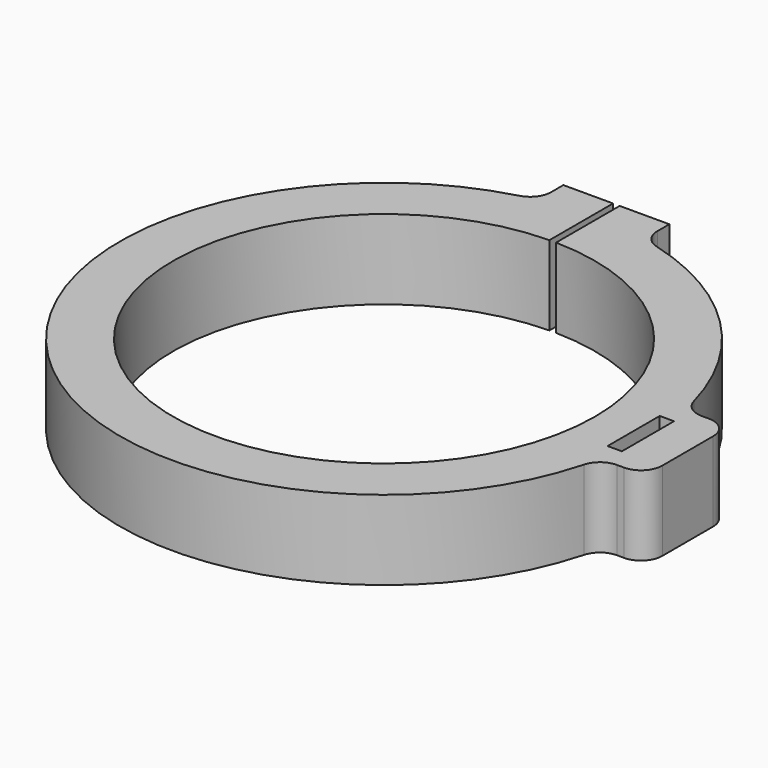
from build123d import *

# Parameters (mm, degrees)
F0_R          = 63.246
F0_R_2        = 50.546
F1_DEPTH      = 19.05
F3_DEPTH      = 19.05
F4_W          = 1.5875
F4_H          = 19.0562327178
F5_DEPTH      = 19.051
F6_R          = 2.5527
F7_DEPTH      = 11.90625
F8_R          = 5.1417133043
F9_DEPTH      = 3.175
F9_DEPTH_BACK = 50.547
F11_D         = 3.7973
F12_W         = 22.225
F12_H         = 25.4
F13_DEPTH     = 19.05
F14_W         = 3.429
F14_H         = 15.621
F15_DEPTH     = 19.0510001
F16_T1_DEPTH  = 19.05
F16_T6_DEPTH  = 14.4190086939
F16_S7_R      = 5.1417133043
F16_T8_DEPTH  = 9
F16_T12_DEPTH = 14.4190086939
F16_S13_R     = 5.1417133043
F16_T14_DEPTH = 9
F16_T18_DEPTH = 17.6620719982
F16_S19_R     = 1.89865
F16_T20_DEPTH = 11
F16_T24_DEPTH = 17.6620719982
F16_S25_R     = 1.89865
F16_T26_DEPTH = 11
F16_T27_DEPTH = 44.45


# Not quite as in the source:
# - a fillet or chamfer that OpenCascade refuses, or shapes differently, is made with other operations: its cross-section is extruded or revolved along the edge and cut away or added


with BuildPart() as f1:
    # F0 (on Top) → F1 (new body)
    with BuildSketch(Plane.XY):
        Circle(F0_R)
        Circle(F0_R_2, mode=Mode.SUBTRACT)
    extrude(amount=F1_DEPTH)

    # F2 (on face) → F3 (join)
    with BuildSketch(Plane.XY.offset(19.05)):
        with BuildLine():
            Line((12.7, 69.596), (-12.7, 69.596))
            Line((-12.7, 69.596), (-12.7, 61.9577801087))
            ThreePointArc((-12.7, 61.9577801087), (0, 63.246), (12.7, 61.9577801087))
            Line((12.7, 61.9577801087), (12.7, 69.596))
        make_face()
    extrude(amount=-F3_DEPTH)

    # F4 (on face) → F5 (cut, through all)
    with BuildSketch(Plane.XY.offset(19.05)):
        with Locations((0, 60.0678836411)):
            Rectangle(F4_W, F4_H)
    extrude(amount=-F5_DEPTH, mode=Mode.SUBTRACT)

    # F6 (on face) → F7 (cut, through all)
    with BuildSketch(Plane.YZ.offset(12.7)):
        with Locations((61.9577801087, 9.525)):
            Circle(F6_R)
    extrude(amount=-F7_DEPTH, mode=Mode.SUBTRACT)

    # F8 (on face) → F9 (cut, two sides)
    with BuildSketch(Plane.YZ.offset(12.7)) as f9_sk:
        with Locations((61.9577801087, 9.525)):
            Circle(F8_R)
    extrude(amount=-F9_DEPTH, mode=Mode.SUBTRACT)
    extrude(f9_sk.sketch, amount=F9_DEPTH_BACK, mode=Mode.SUBTRACT)

    # F11 (through all)
    with Locations(Plane.YZ.offset(-0.79375)):
        with Locations((61.9577801087, 9.525)):
            Hole(F11_D / 2)

    # F12 (on face) → F13 (join)
    with BuildSketch(Plane.XY.offset(19.05)):
        with Locations((61.6585, 0)):
            Rectangle(F12_W, F12_H)
    extrude(amount=-F13_DEPTH)

    # F14 (on face) → F15 (cut, through all)
    with BuildSketch(Plane.XY.offset(19.05)):
        with Locations((61.5315, 0)):
            Rectangle(F14_W, F14_H)
    extrude(amount=-F15_DEPTH, mode=Mode.SUBTRACT)

    # F16: fillet of radius 5.08 on 8 edges, made by hand

    # F16_s2 → F16_t1 (join)
    with BuildSketch(Plane.XY):
        with BuildLine():
            ThreePointArc((61.0670823721, -16.4580669145), (62.882491273, -13.7475181293), (65.972068908, -12.7))
            Line((65.972068908, -12.7), (61.9577801087, -12.7))
            ThreePointArc((61.9577801087, -12.7), (61.5411241678, -14.585833955), (61.0670823721, -16.4580669145))
        make_face()
        with BuildLine():
            ThreePointArc((65.972068908, 12.7), (62.882491273, 13.7475181293), (61.0670823721, 16.4580669145))
            ThreePointArc((61.0670823721, 16.4580669145), (61.5411241678, 14.585833955), (61.9577801087, 12.7))
            Line((61.9577801087, 12.7), (65.972068908, 12.7))
        make_face()
    extrude(amount=F16_T1_DEPTH)


with BuildPart() as f16_tool4:
    # F16_s5 → F16_t6 (new body)
    with BuildSketch(Plane.XY.offset(19.05)):
        with BuildLine():
            ThreePointArc((16.4580669145, 61.0670823721), (13.7475181293, 62.882491273), (12.7, 65.972068908))
            Line((12.7, 65.972068908), (12.7, 61.9577801087))
            ThreePointArc((12.7, 61.9577801087), (14.585833955, 61.5411241678), (16.4580669145, 61.0670823721))
        make_face()
    extrude(amount=-F16_T6_DEPTH)

    # F16_s7 → F16_t8 (cut, symmetric)
    with BuildSketch(Plane.YZ.offset(14.6)):
        with Locations((61.9577801087, 9.525)):
            Circle(F16_S7_R)
    extrude(amount=F16_T8_DEPTH, both=True, mode=Mode.SUBTRACT)


with BuildPart() as f1_1:
    add(f1.part)

    # F16_t3: union F16_tool4
    add(f16_tool4.part)


with BuildPart() as f16_tool10:
    # F16_s11 → F16_t12 (new body)
    with BuildSketch(Plane.XY.offset(14.4190086939)):
        with BuildLine():
            ThreePointArc((16.4580669145, 61.0670823721), (13.7475181293, 62.882491273), (12.7, 65.972068908))
            Line((12.7, 65.972068908), (12.7, 61.9577801087))
            ThreePointArc((12.7, 61.9577801087), (14.585833955, 61.5411241678), (16.4580669145, 61.0670823721))
        make_face()
    extrude(amount=-F16_T12_DEPTH)

    # F16_s13 → F16_t14 (cut, symmetric)
    with BuildSketch(Plane.YZ.offset(14.6)):
        with Locations((61.9577801087, 9.525)):
            Circle(F16_S13_R)
    extrude(amount=F16_T14_DEPTH, both=True, mode=Mode.SUBTRACT)


with BuildPart() as f1_2:
    add(f1_1.part)

    # F16_t9: union F16_tool10
    add(f16_tool10.part)


with BuildPart() as f16_tool16:
    # F16_s17 → F16_t18 (new body)
    with BuildSketch(Plane.XY.offset(19.05)):
        with BuildLine():
            ThreePointArc((-16.4580669145, 61.0670823721), (-13.7475181293, 62.882491273), (-12.7, 65.972068908))
            Line((-12.7, 65.972068908), (-12.7, 61.9577801087))
            ThreePointArc((-12.7, 61.9577801087), (-14.585833955, 61.5411241678), (-16.4580669145, 61.0670823721))
        make_face()
    extrude(amount=-F16_T18_DEPTH)

    # F16_s19 → F16_t20 (cut, symmetric)
    with BuildSketch(Plane.YZ.offset(-14.6)):
        with Locations((61.9577801087, 9.525)):
            Circle(F16_S19_R)
    extrude(amount=F16_T20_DEPTH, both=True, mode=Mode.SUBTRACT)


with BuildPart() as f1_3:
    add(f1_2.part)

    # F16_t15: union F16_tool16
    add(f16_tool16.part)


with BuildPart() as f16_tool22:
    # F16_s23 → F16_t24 (new body)
    with BuildSketch(Plane.XY.offset(17.6620719982)):
        with BuildLine():
            ThreePointArc((-16.4580669145, 61.0670823721), (-13.7475181293, 62.882491273), (-12.7, 65.972068908))
            Line((-12.7, 65.972068908), (-12.7, 61.9577801087))
            ThreePointArc((-12.7, 61.9577801087), (-14.585833955, 61.5411241678), (-16.4580669145, 61.0670823721))
        make_face()
    extrude(amount=-F16_T24_DEPTH)

    # F16_s25 → F16_t26 (cut, symmetric)
    with BuildSketch(Plane.YZ.offset(-14.6)):
        with Locations((61.9577801087, 9.525)):
            Circle(F16_S25_R)
    extrude(amount=F16_T26_DEPTH, both=True, mode=Mode.SUBTRACT)


with BuildPart() as f1_4:
    add(f1_3.part)

    # F16_t21: union F16_tool22
    add(f16_tool22.part)

    # F16_s28 → F16_t27 (cut)
    with BuildSketch(Plane.XY.offset(-12.7)):
        with BuildLine():
            ThreePointArc((67.691, -12.7), (71.2831024484, -11.2121024484), (72.771, -7.62))
            Line((72.771, -7.62), (72.771, -12.7))
            Line((72.771, -12.7), (67.691, -12.7))
        make_face()
        with BuildLine():
            ThreePointArc((72.771, 7.62), (71.2831024484, 11.2121024484), (67.691, 12.7))
            Line((67.691, 12.7), (72.771, 12.7))
            Line((72.771, 12.7), (72.771, 7.62))
        make_face()
    extrude(amount=F16_T27_DEPTH, mode=Mode.SUBTRACT)


solid = f1_4.part
